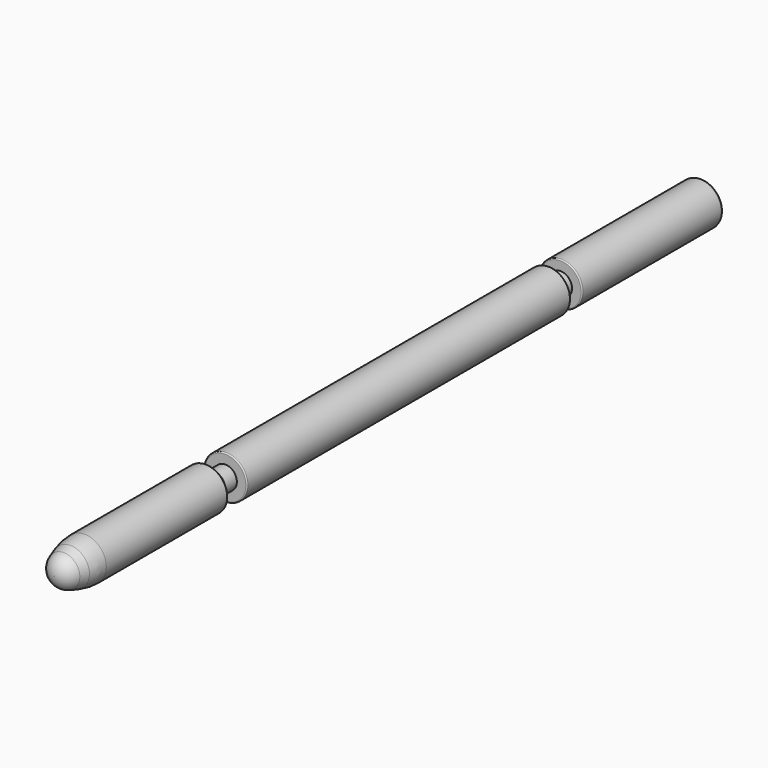
from build123d import *

# Parameters (mm, degrees)
F0_R        = 2.38125
F1_DEPTH    = 88.9
F2_SIZE2    = 3.175
F2_SIZE     = 1.016
F3_R        = 1.8542
F4_R        = 6.35
F5_R        = 0.254
F6_W        = 3.5311071049
F6_H        = 1.5875
F8_S5_R     = 1.27
F8_T6_DEPTH = 5
F9_R        = 0.127


# Not quite as in the source:
# - a fillet or chamfer that OpenCascade refuses, or shapes differently, is made with other operations: its cross-section is extruded or revolved along the edge and cut away or added


with BuildPart() as f1:
    # F0 (on Front) → F1 (new body)
    with BuildSketch(Plane.XZ):
        Circle(F0_R)
    extrude(amount=F1_DEPTH)

    # F2
    f2_edges = [f1.edges().sort_by_distance(p)[0] for p in [
        (-2.38125, -88.9, 0),
    ]]
    f2_side = f1.faces().sort_by_distance((0, -88.9, 0))[0]
    chamfer(f2_edges, length=F2_SIZE, length2=F2_SIZE2, reference=f2_side)

    # F3
    f3_edges = [f1.edges().sort_by_distance(p)[0] for p in [
        (-1.36525, -88.9, 0),
    ]]
    fillet(f3_edges, radius=F3_R)

    # F4
    f4_edges = [f1.edges().sort_by_distance(p)[0] for p in [
        (-2.38125, -85.725, 0),
    ]]
    fillet(f4_edges, radius=F4_R)

    # F5
    f5_edges = [f1.edges().sort_by_distance(p)[0] for p in [
        (-2.38125, 0, 0),
    ]]
    fillet(f5_edges, radius=F5_R)

    # F6 (on Top) → F7 (revolve, cut)
    with BuildSketch(Plane.XY):
        with Locations((3.0355535524, -20.16125)):
            Rectangle(F6_W, F6_H)
        with Locations((3.0355535524, -66.19875)):
            Rectangle(F6_W, F6_H)
    revolve(axis=Axis((0, -11.8038663641, 0), (0, -1, 0)), mode=Mode.SUBTRACT)

    # F8: chamfer of 1.1176 on 1 edges, made by hand


with BuildPart() as f8_tool2:
    # F8_s3 → F8_t4 (revolve)
    with BuildSketch(Plane.XY):
        Polygon((1.26365, -66.9925), (2.38125, -68.1101), (2.38125, -66.9925), align=None)
    revolve(axis=Axis((0, -66.9925, 0), (0, 1, 0)))

    # F8_s5 → F8_t6 (cut, symmetric)
    with BuildSketch(Plane.XZ.offset(67.6)):
        Circle(F8_S5_R)
    extrude(amount=F8_T6_DEPTH, both=True, mode=Mode.SUBTRACT)


with BuildPart() as f1_1:
    add(f1.part)

    # F8_t1: cut F8_tool2
    add(f8_tool2.part, mode=Mode.SUBTRACT)

    # F9
    f9_edges = [f1_1.edges().sort_by_distance(p)[0] for p in [
        (-2.38125, -19.3675, 0),
        (-2.38125, -20.955, 0),
        (-2.38125, -65.405, 0),
        (-2.38125, -68.1101, 0),
    ]]
    fillet(f9_edges, radius=F9_R)


solid = f1_1.part
